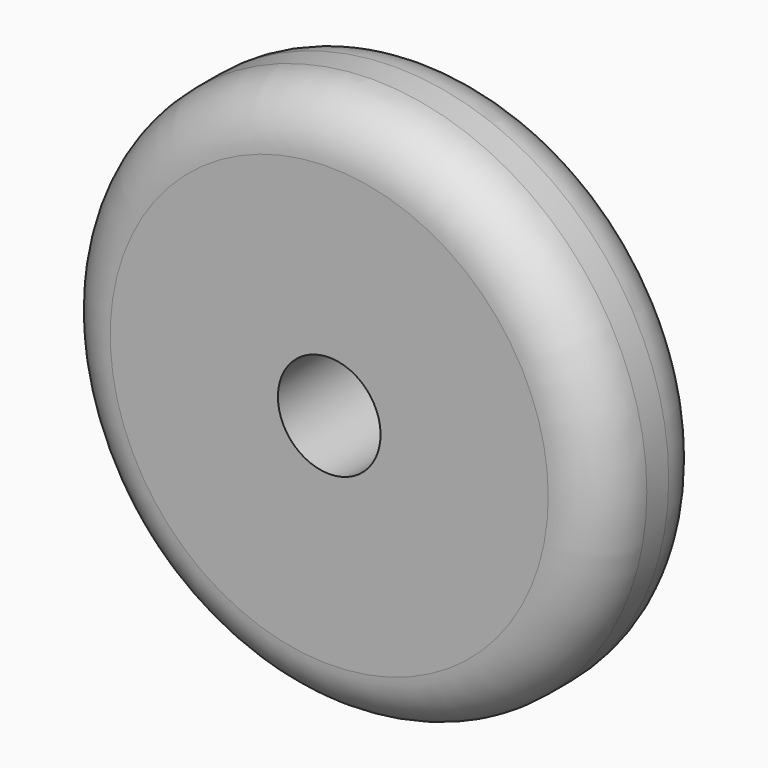
from build123d import *

# Parameters (mm, degrees)
F1_DEPTH = 6.35


# Not quite as in the source:
# - a fillet or chamfer that OpenCascade refuses, or shapes differently, is made with other operations: its cross-section is extruded or revolved along the edge and cut away or added


with BuildPart() as f1:
    # F0 (on Front) → F1 (new body)
    with BuildSketch(Plane.XZ):
        with BuildLine():
            ThreePointArc((12.7, 0), (0, 12.7), (-12.7, 0))
            ThreePointArc((-12.7, 0), (0, -12.7), (12.7, 0))
        make_face()
        with BuildLine():
            ThreePointArc((0, -2.38125), (-1.6837980227, -1.6837980227), (-2.38125, 0))
            ThreePointArc((-2.38125, 0), (0, 2.38125), (2.38125, 0))
            ThreePointArc((2.38125, 0), (1.6837980227, -1.6837980227), (0, -2.38125))
        make_face(mode=Mode.SUBTRACT)
    extrude(amount=F1_DEPTH)

    # F2: fillet of radius 2.54 on 2 edges, made by hand

    # F2_s1 → F2_t2 (revolve, cut)
    with BuildSketch(Plane.XY):
        with BuildLine():
            ThreePointArc((12.7, -3.81), (11.9560512242, -5.6060512242), (10.16, -6.35))
            Line((10.16, -6.35), (12.7, -6.35))
            Line((12.7, -6.35), (12.7, -3.81))
        make_face()
    revolve(axis=Axis((0, -6.35, 0), (0, 1, 0)), mode=Mode.SUBTRACT)

    # F2_s3 → F2_t4 (revolve, cut)
    with BuildSketch(Plane.XY):
        with BuildLine():
            ThreePointArc((12.7, -2.54), (11.9560512242, -0.7439487758), (10.16, 0))
            Line((10.16, 0), (12.7, 0))
            Line((12.7, 0), (12.7, -2.54))
        make_face()
    revolve(axis=Axis((0, 0, 0), (0, -1, 0)), mode=Mode.SUBTRACT)


solid = f1.part
